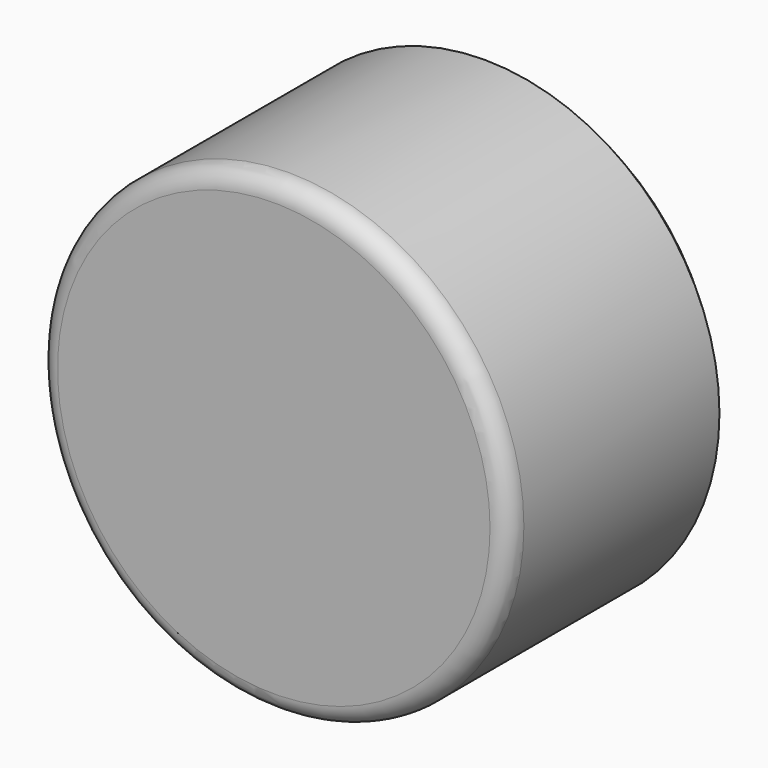
from build123d import *

# Parameters (mm, degrees)
F0_R     = 63.5
F1_DEPTH = 76.2
F6_R     = 5.08
F7_SIZE  = 5.08


# Not quite as in the source:
# - the program builds the solid bodies; features that only make, move or delete a surface that nothing else refers to are left out


with BuildPart() as f1:
    # F0 (on Front) → F1 (new body)
    with BuildSketch(Plane.XZ):
        Circle(F0_R)
    extrude(amount=F1_DEPTH)

    # F6
    f6_edges = [f1.edges().sort_by_distance(p)[0] for p in [
        (-63.5, -76.2, 0),
    ]]
    fillet(f6_edges, radius=F6_R)

    # F7
    f7_edges = [f1.edges().sort_by_distance(p)[0] for p in [
        (-63.5, 0, 0),
    ]]
    chamfer(f7_edges, length=F7_SIZE)


solid = f1.part
